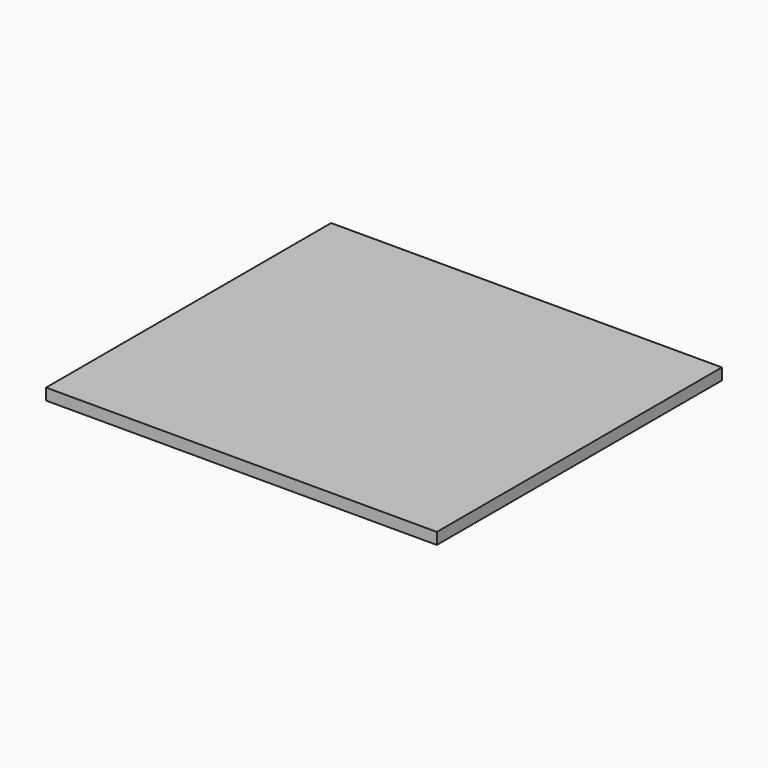
from build123d import *

# Parameters (mm, degrees)
F0_W     = 53.975
F0_H     = 49.2125
F1_DEPTH = 1.5875


# Not quite as in the source:
# - a feature of the source that left no trace in its solid (it failed there, or was rolled back) is left out


with BuildPart() as f1:
    # F0 (on Top) → F1 (new body)
    with BuildSketch(Plane.XY):
        with Locations((0, 8.73125)):
            Rectangle(F0_W, F0_H)
    extrude(amount=F1_DEPTH)


solid = f1.part
